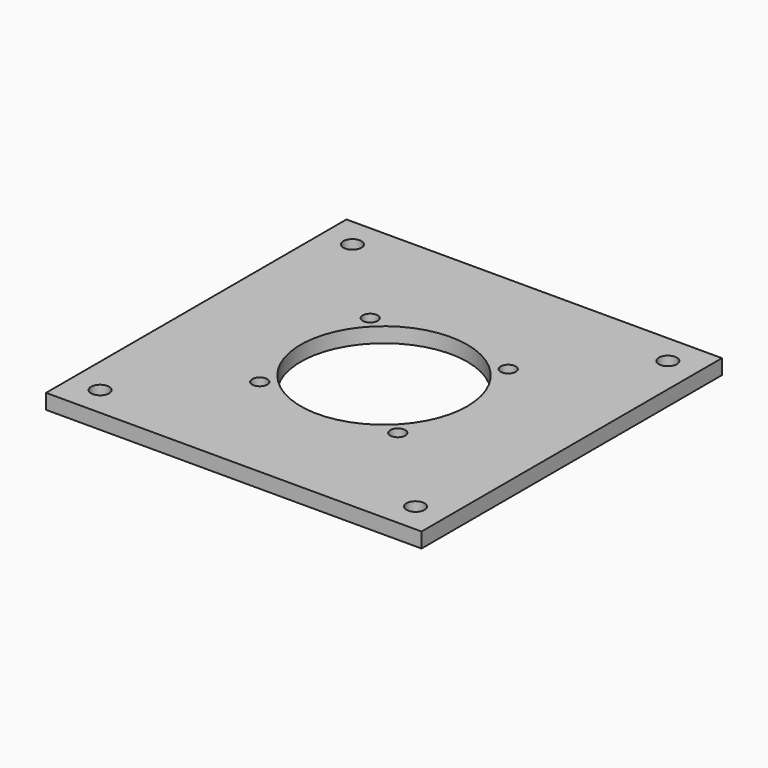
from build123d import *

# Parameters (mm, degrees)
F0_W            = 250
F0_H            = 250
F0_R            = 55.5
F1_DEPTH        = 10
F2_R            = 5
F3_DEPTH        = 25
F3_COPIES_COUNT = 4
F4_R            = 6
F5_DEPTH        = 10.001


# Not quite as in the source:
# - a pattern or mirror of a feature is missing from the dataset's text; its kind, count and spacing are read off the source's solid


with BuildPart() as f1:
    # F0 (on Top) → F1 (new body)
    with BuildSketch(Plane.XY):
        Rectangle(F0_W, F0_H)
        Circle(F0_R, mode=Mode.SUBTRACT)
    extrude(amount=F1_DEPTH)

    # F2 (on face) → F3 (cut)
    with BuildSketch(Plane.XY.offset(10)):
        with Locations((-45.9619407771, 45.9619407771)):
            Circle(F2_R)
    f3 = extrude(amount=-F3_DEPTH, mode=Mode.SUBTRACT)

    # F3_copies: F3 ×4 about axis
    f3_copies_axis = Axis((0, 0, 0), (0, 0, 1))
    for i in range(1, F3_COPIES_COUNT):
        add(f3.rotate(f3_copies_axis, i * 360 / F3_COPIES_COUNT), mode=Mode.SUBTRACT)

    # F4 (on face) → F5 (cut, through all)
    with BuildSketch(Plane.XY.offset(10)):
        with Locations((-105, 105)):
            Circle(F4_R)
        with Locations((105, 105)):
            Circle(F4_R)
        with Locations((105, -105)):
            Circle(F4_R)
        with Locations((-105, -105)):
            Circle(F4_R)
    extrude(amount=-F5_DEPTH, mode=Mode.SUBTRACT)


solid = f1.part
